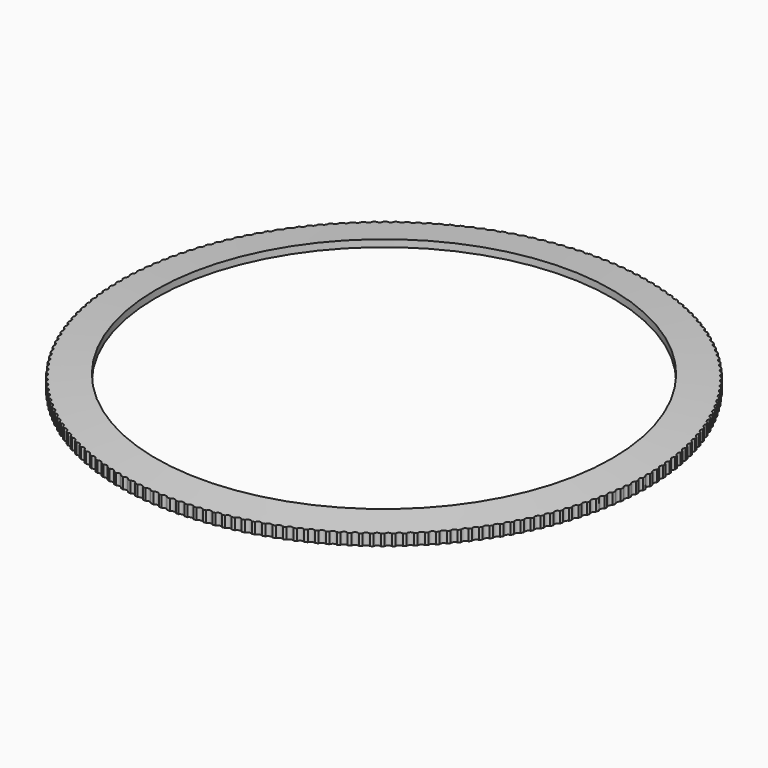
from build123d import *

# Parameters (mm, degrees)
F3_R      = 18.215
F3_R_2    = 16.85
F6_DEPTH  = 1.2
F3_R_3    = 15.75
F7_DEPTH  = 0.7
F9_R      = 0.25
F10_DEPTH = 1.2


# Not quite as in the source:
# - a fillet or chamfer that OpenCascade refuses, or shapes differently, is made with other operations: its cross-section is extruded or revolved along the edge and cut away or added


with BuildPart() as f6:
    # F3 (on Top) → F6 (new body)
    with BuildSketch(Plane.XY):
        Circle(F3_R)
        Circle(F3_R_2, mode=Mode.SUBTRACT)
    extrude(amount=-F6_DEPTH)

    # F3 (on Top) → F7 (join)
    with BuildSketch(Plane.XY):
        Circle(F3_R_2)
        Circle(F3_R_3, mode=Mode.SUBTRACT)
    extrude(amount=-F7_DEPTH)

    # F8: chamfer of 4.93 x 0.4313191112 on 1 edges, made by hand

    # F8_s1 → F8_t2 (revolve, cut)
    with BuildSketch(Plane.XZ):
        Polygon((18.215, -0.4313191112), (13.285, 0), (18.215, 0), align=None)
    revolve(axis=Axis((0, 0, 0), (0, 0, 1)), mode=Mode.SUBTRACT)

    # F9 (on Top) → F10 (cut)
    with BuildSketch(Plane.XY):
        with Locations((0, 18.365)):
            Circle(F9_R)
        with Locations((-0.600885956, 18.355167149)):
            Circle(F9_R)
        with Locations((-1.2011284683, 18.3256791253)):
            Circle(F9_R)
        with Locations((-1.8000847822, 18.2765675053)):
            Circle(F9_R)
        with Locations((-2.3971135201, 18.2078848791)):
            Circle(F9_R)
        with Locations((-2.9915753689, 18.1197047937)):
            Circle(F9_R)
        with Locations((-3.5828337638, 18.0121216746)):
            Circle(F9_R)
        with Locations((-4.1702555706, 17.8852507244)):
            Circle(F9_R)
        with Locations((-4.7532117633, 17.7392277998)):
            Circle(F9_R)
        with Locations((-5.3310780978, 17.5742092657)):
            Circle(F9_R)
        with Locations((-5.9032357803, 17.3903718282)):
            Circle(F9_R)
        with Locations((-6.4690721301, 17.1879123449)):
            Circle(F9_R)
        with Locations((-7.0279812354, 16.9670476146)):
            Circle(F9_R)
        with Locations((-7.5793646024, 16.7280141447)):
            Circle(F9_R)
        with Locations((-8.1226317959, 16.4710678982)):
            Circle(F9_R)
        with Locations((-8.6572010718, 16.1964840198)):
            Circle(F9_R)
        with Locations((-9.1825, 15.9045565405)):
            Circle(F9_R)
        with Locations((-9.6979660772, 15.5955980637)):
            Circle(F9_R)
        with Locations((-10.2030473294, 15.2699394299)):
            Circle(F9_R)
        with Locations((-10.697202903, 14.9279293625)):
            Circle(F9_R)
        with Locations((-11.1799036437, 14.5699340944)):
            Circle(F9_R)
        with Locations((-11.6506326637, 14.196336976)):
            Circle(F9_R)
        with Locations((-12.1088858943, 13.8075380644)):
            Circle(F9_R)
        with Locations((-12.5541726267, 13.4039536951)):
            Circle(F9_R)
        with Locations((-12.9860160365, 12.9860160365)):
            Circle(F9_R)
        with Locations((-13.4039536951, 12.5541726267)):
            Circle(F9_R)
        with Locations((-13.8075380644, 12.1088858943)):
            Circle(F9_R)
        with Locations((-14.196336976, 11.6506326637)):
            Circle(F9_R)
        with Locations((-14.5699340944, 11.1799036437)):
            Circle(F9_R)
        with Locations((-14.9279293625, 10.697202903)):
            Circle(F9_R)
        with Locations((-15.2699394299, 10.2030473294)):
            Circle(F9_R)
        with Locations((-15.5955980637, 9.6979660772)):
            Circle(F9_R)
        with Locations((-15.9045565405, 9.1825)):
            Circle(F9_R)
        with Locations((-16.1964840198, 8.6572010718)):
            Circle(F9_R)
        with Locations((-16.4710678982, 8.1226317959)):
            Circle(F9_R)
        with Locations((-16.7280141447, 7.5793646024)):
            Circle(F9_R)
        with Locations((-16.9670476146, 7.0279812354)):
            Circle(F9_R)
        with Locations((-17.1879123449, 6.4690721301)):
            Circle(F9_R)
        with Locations((-17.3903718282, 5.9032357803)):
            Circle(F9_R)
        with Locations((-17.5742092657, 5.3310780978)):
            Circle(F9_R)
        with Locations((-17.7392277998, 4.7532117633)):
            Circle(F9_R)
        with Locations((-17.8852507244, 4.1702555706)):
            Circle(F9_R)
        with Locations((-18.0121216746, 3.5828337638)):
            Circle(F9_R)
        with Locations((-18.1197047937, 2.9915753689)):
            Circle(F9_R)
        with Locations((-18.2078848791, 2.3971135201)):
            Circle(F9_R)
        with Locations((-18.2765675053, 1.8000847822)):
            Circle(F9_R)
        with Locations((-18.3256791253, 1.2011284683)):
            Circle(F9_R)
        with Locations((-18.355167149, 0.600885956)):
            Circle(F9_R)
        with Locations((-18.365, 0)):
            Circle(F9_R)
        with Locations((-18.355167149, -0.600885956)):
            Circle(F9_R)
        with Locations((-18.3256791253, -1.2011284683)):
            Circle(F9_R)
        with Locations((-18.2765675053, -1.8000847822)):
            Circle(F9_R)
        with Locations((-18.2078848791, -2.3971135201)):
            Circle(F9_R)
        with Locations((-18.1197047937, -2.9915753689)):
            Circle(F9_R)
        with Locations((-18.0121216746, -3.5828337638)):
            Circle(F9_R)
        with Locations((-17.8852507244, -4.1702555706)):
            Circle(F9_R)
        with Locations((-17.7392277998, -4.7532117633)):
            Circle(F9_R)
        with Locations((-17.5742092657, -5.3310780978)):
            Circle(F9_R)
        with Locations((-17.3903718282, -5.9032357803)):
            Circle(F9_R)
        with Locations((-17.1879123449, -6.4690721301)):
            Circle(F9_R)
        with Locations((-16.9670476146, -7.0279812354)):
            Circle(F9_R)
        with Locations((-16.7280141447, -7.5793646024)):
            Circle(F9_R)
        with Locations((-16.4710678982, -8.1226317959)):
            Circle(F9_R)
        with Locations((-16.1964840198, -8.6572010718)):
            Circle(F9_R)
        with Locations((-15.9045565405, -9.1825)):
            Circle(F9_R)
        with Locations((-15.5955980637, -9.6979660772)):
            Circle(F9_R)
        with Locations((-15.2699394299, -10.2030473294)):
            Circle(F9_R)
        with Locations((-14.9279293625, -10.697202903)):
            Circle(F9_R)
        with Locations((-14.5699340944, -11.1799036437)):
            Circle(F9_R)
        with Locations((-14.196336976, -11.6506326637)):
            Circle(F9_R)
        with Locations((-13.8075380644, -12.1088858943)):
            Circle(F9_R)
        with Locations((-13.4039536951, -12.5541726267)):
            Circle(F9_R)
        with Locations((-12.9860160365, -12.9860160365)):
            Circle(F9_R)
        with Locations((-12.5541726267, -13.4039536951)):
            Circle(F9_R)
        with Locations((-12.1088858943, -13.8075380644)):
            Circle(F9_R)
        with Locations((-11.6506326637, -14.196336976)):
            Circle(F9_R)
        with Locations((-11.1799036437, -14.5699340944)):
            Circle(F9_R)
        with Locations((-10.697202903, -14.9279293625)):
            Circle(F9_R)
        with Locations((-10.2030473294, -15.2699394299)):
            Circle(F9_R)
        with Locations((-9.6979660772, -15.5955980637)):
            Circle(F9_R)
        with Locations((-9.1825, -15.9045565405)):
            Circle(F9_R)
        with Locations((-8.6572010718, -16.1964840198)):
            Circle(F9_R)
        with Locations((-8.1226317959, -16.4710678982)):
            Circle(F9_R)
        with Locations((-7.5793646024, -16.7280141447)):
            Circle(F9_R)
        with Locations((-7.0279812354, -16.9670476146)):
            Circle(F9_R)
        with Locations((-6.4690721301, -17.1879123449)):
            Circle(F9_R)
        with Locations((-5.9032357803, -17.3903718282)):
            Circle(F9_R)
        with Locations((-5.3310780978, -17.5742092657)):
            Circle(F9_R)
        with Locations((-4.7532117633, -17.7392277998)):
            Circle(F9_R)
        with Locations((-4.1702555706, -17.8852507244)):
            Circle(F9_R)
        with Locations((-3.5828337638, -18.0121216746)):
            Circle(F9_R)
        with Locations((-2.9915753689, -18.1197047937)):
            Circle(F9_R)
        with Locations((-2.3971135201, -18.2078848791)):
            Circle(F9_R)
        with Locations((-1.8000847822, -18.2765675053)):
            Circle(F9_R)
        with Locations((-1.2011284683, -18.3256791253)):
            Circle(F9_R)
        with Locations((-0.600885956, -18.355167149)):
            Circle(F9_R)
        with Locations((0, -18.365)):
            Circle(F9_R)
        with Locations((0.600885956, -18.355167149)):
            Circle(F9_R)
        with Locations((1.2011284683, -18.3256791253)):
            Circle(F9_R)
        with Locations((1.8000847822, -18.2765675053)):
            Circle(F9_R)
        with Locations((2.3971135201, -18.2078848791)):
            Circle(F9_R)
        with Locations((2.9915753689, -18.1197047937)):
            Circle(F9_R)
        with Locations((3.5828337638, -18.0121216746)):
            Circle(F9_R)
        with Locations((4.1702555706, -17.8852507244)):
            Circle(F9_R)
        with Locations((4.7532117633, -17.7392277998)):
            Circle(F9_R)
        with Locations((5.3310780978, -17.5742092657)):
            Circle(F9_R)
        with Locations((5.9032357803, -17.3903718282)):
            Circle(F9_R)
        with Locations((6.4690721301, -17.1879123449)):
            Circle(F9_R)
        with Locations((7.0279812354, -16.9670476146)):
            Circle(F9_R)
        with Locations((7.5793646024, -16.7280141447)):
            Circle(F9_R)
        with Locations((8.1226317959, -16.4710678982)):
            Circle(F9_R)
        with Locations((8.6572010718, -16.1964840198)):
            Circle(F9_R)
        with Locations((9.1825, -15.9045565405)):
            Circle(F9_R)
        with Locations((9.6979660772, -15.5955980637)):
            Circle(F9_R)
        with Locations((10.2030473294, -15.2699394299)):
            Circle(F9_R)
        with Locations((10.697202903, -14.9279293625)):
            Circle(F9_R)
        with Locations((11.1799036437, -14.5699340944)):
            Circle(F9_R)
        with Locations((11.6506326637, -14.196336976)):
            Circle(F9_R)
        with Locations((12.1088858943, -13.8075380644)):
            Circle(F9_R)
        with Locations((12.5541726267, -13.4039536951)):
            Circle(F9_R)
        with Locations((12.9860160365, -12.9860160365)):
            Circle(F9_R)
        with Locations((13.4039536951, -12.5541726267)):
            Circle(F9_R)
        with Locations((13.8075380644, -12.1088858943)):
            Circle(F9_R)
        with Locations((14.196336976, -11.6506326637)):
            Circle(F9_R)
        with Locations((14.5699340944, -11.1799036437)):
            Circle(F9_R)
        with Locations((14.9279293625, -10.697202903)):
            Circle(F9_R)
        with Locations((15.2699394299, -10.2030473294)):
            Circle(F9_R)
        with Locations((15.5955980637, -9.6979660772)):
            Circle(F9_R)
        with Locations((15.9045565405, -9.1825)):
            Circle(F9_R)
        with Locations((16.1964840198, -8.6572010718)):
            Circle(F9_R)
        with Locations((16.4710678982, -8.1226317959)):
            Circle(F9_R)
        with Locations((16.7280141447, -7.5793646024)):
            Circle(F9_R)
        with Locations((16.9670476146, -7.0279812354)):
            Circle(F9_R)
        with Locations((17.1879123449, -6.4690721301)):
            Circle(F9_R)
        with Locations((17.3903718282, -5.9032357803)):
            Circle(F9_R)
        with Locations((17.5742092657, -5.3310780978)):
            Circle(F9_R)
        with Locations((17.7392277998, -4.7532117633)):
            Circle(F9_R)
        with Locations((17.8852507244, -4.1702555706)):
            Circle(F9_R)
        with Locations((18.0121216746, -3.5828337638)):
            Circle(F9_R)
        with Locations((18.1197047937, -2.9915753689)):
            Circle(F9_R)
        with Locations((18.2078848791, -2.3971135201)):
            Circle(F9_R)
        with Locations((18.2765675053, -1.8000847822)):
            Circle(F9_R)
        with Locations((18.3256791253, -1.2011284683)):
            Circle(F9_R)
        with Locations((18.355167149, -0.600885956)):
            Circle(F9_R)
        with Locations((18.365, 0)):
            Circle(F9_R)
        with Locations((18.355167149, 0.600885956)):
            Circle(F9_R)
        with Locations((18.3256791253, 1.2011284683)):
            Circle(F9_R)
        with Locations((18.2765675053, 1.8000847822)):
            Circle(F9_R)
        with Locations((18.2078848791, 2.3971135201)):
            Circle(F9_R)
        with Locations((18.1197047937, 2.9915753689)):
            Circle(F9_R)
        with Locations((18.0121216746, 3.5828337638)):
            Circle(F9_R)
        with Locations((17.8852507244, 4.1702555706)):
            Circle(F9_R)
        with Locations((17.7392277998, 4.7532117633)):
            Circle(F9_R)
        with Locations((17.5742092657, 5.3310780978)):
            Circle(F9_R)
        with Locations((17.3903718282, 5.9032357803)):
            Circle(F9_R)
        with Locations((17.1879123449, 6.4690721301)):
            Circle(F9_R)
        with Locations((16.9670476146, 7.0279812354)):
            Circle(F9_R)
        with Locations((16.7280141447, 7.5793646024)):
            Circle(F9_R)
        with Locations((16.4710678982, 8.1226317959)):
            Circle(F9_R)
        with Locations((16.1964840198, 8.6572010718)):
            Circle(F9_R)
        with Locations((15.9045565405, 9.1825)):
            Circle(F9_R)
        with Locations((15.5955980637, 9.6979660772)):
            Circle(F9_R)
        with Locations((15.2699394299, 10.2030473294)):
            Circle(F9_R)
        with Locations((14.9279293625, 10.697202903)):
            Circle(F9_R)
        with Locations((14.5699340944, 11.1799036437)):
            Circle(F9_R)
        with Locations((14.196336976, 11.6506326637)):
            Circle(F9_R)
        with Locations((13.8075380644, 12.1088858943)):
            Circle(F9_R)
        with Locations((13.4039536951, 12.5541726267)):
            Circle(F9_R)
        with Locations((12.9860160365, 12.9860160365)):
            Circle(F9_R)
        with Locations((12.5541726267, 13.4039536951)):
            Circle(F9_R)
        with Locations((12.1088858943, 13.8075380644)):
            Circle(F9_R)
        with Locations((11.6506326637, 14.196336976)):
            Circle(F9_R)
        with Locations((11.1799036437, 14.5699340944)):
            Circle(F9_R)
        with Locations((10.697202903, 14.9279293625)):
            Circle(F9_R)
        with Locations((10.2030473294, 15.2699394299)):
            Circle(F9_R)
        with Locations((9.6979660772, 15.5955980637)):
            Circle(F9_R)
        with Locations((9.1825, 15.9045565405)):
            Circle(F9_R)
        with Locations((8.6572010718, 16.1964840198)):
            Circle(F9_R)
        with Locations((8.1226317959, 16.4710678982)):
            Circle(F9_R)
        with Locations((7.5793646024, 16.7280141447)):
            Circle(F9_R)
        with Locations((7.0279812354, 16.9670476146)):
            Circle(F9_R)
        with Locations((6.4690721301, 17.1879123449)):
            Circle(F9_R)
        with Locations((5.9032357803, 17.3903718282)):
            Circle(F9_R)
        with Locations((5.3310780978, 17.5742092657)):
            Circle(F9_R)
        with Locations((4.7532117633, 17.7392277998)):
            Circle(F9_R)
        with Locations((4.1702555706, 17.8852507244)):
            Circle(F9_R)
        with Locations((3.5828337638, 18.0121216746)):
            Circle(F9_R)
        with Locations((2.9915753689, 18.1197047937)):
            Circle(F9_R)
        with Locations((2.3971135201, 18.2078848791)):
            Circle(F9_R)
        with Locations((1.8000847822, 18.2765675053)):
            Circle(F9_R)
        with Locations((1.2011284683, 18.3256791253)):
            Circle(F9_R)
        with Locations((0.600885956, 18.355167149)):
            Circle(F9_R)
    extrude(amount=-F10_DEPTH, mode=Mode.SUBTRACT)


solid = f6.part
